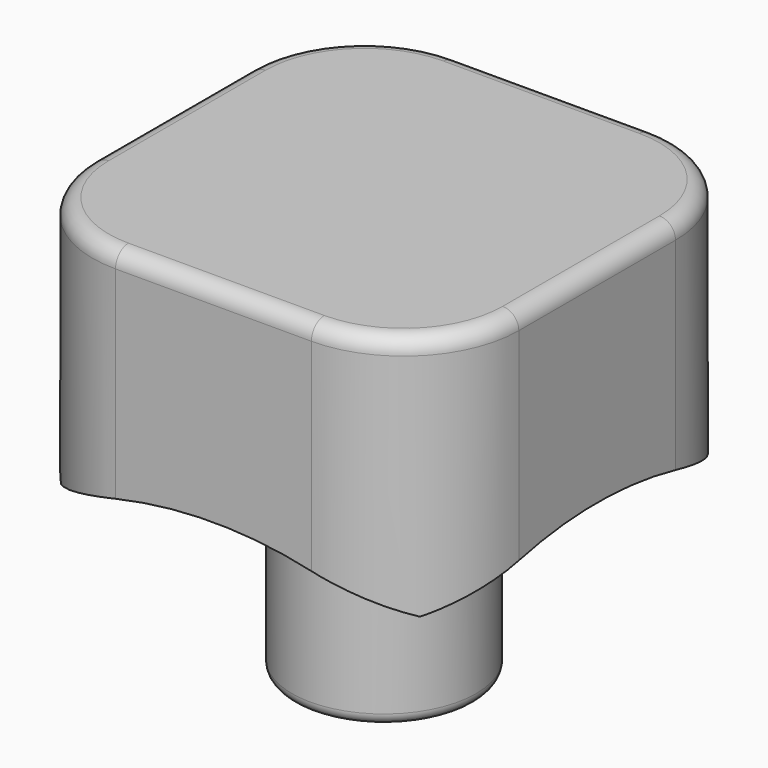
from build123d import *

# Parameters (mm, degrees)
F0_W         = 18.5
F0_H         = 11
F1_DEPTH     = 9.25
F2_DEPTH     = 9.25
F3_R         = 19
F5_DEPTH     = 25.4
F6_DEPTH     = 25.4
F4_R         = 19
F7_DEPTH     = 25.4
F8_DEPTH     = 25.4
F9_R         = 4
F10_DEPTH    = 3.45753
F11_DEPTH    = 7.5
F12_T1_DEPTH = 36
F13_R        = 0.7
F14_R        = 0.5


# Not quite as in the source:
# - a fillet or chamfer that OpenCascade refuses, or shapes differently, is made with other operations: its cross-section is extruded or revolved along the edge and cut away or added
# - a feature names something its author has since deleted; it is built from what else it names


with BuildPart() as f1:
    # F0 (on Front) → F1 (new body)
    with BuildSketch(Plane.XZ):
        Rectangle(F0_W, F0_H)
    extrude(amount=-F1_DEPTH)

    # F0 (on Front) → F2 (join)
    with BuildSketch(Plane.XZ):
        Rectangle(F0_W, F0_H)
    extrude(amount=F2_DEPTH)

    # F3 (on Front) → F5 (cut)
    with BuildSketch(Plane.XZ):
        with Locations((0, -22.5)):
            Circle(F3_R)
    extrude(amount=-F5_DEPTH, mode=Mode.SUBTRACT)

    # F3 (on Front) → F6 (cut)
    with BuildSketch(Plane.XZ):
        with Locations((0, -22.5)):
            Circle(F3_R)
    extrude(amount=F6_DEPTH, mode=Mode.SUBTRACT)

    # F4 (on Right) → F7 (cut)
    with BuildSketch(Plane.YZ):
        with Locations((0, -22.5)):
            Circle(F4_R)
    extrude(amount=-F7_DEPTH, mode=Mode.SUBTRACT)

    # F4 (on Right) → F8 (cut)
    with BuildSketch(Plane.YZ):
        with Locations((0, -22.5)):
            Circle(F4_R)
    extrude(amount=F8_DEPTH, mode=Mode.SUBTRACT)

    # F9 (on face) → F10 (join)
    with BuildSketch(Plane(origin=(0, 0, -5.5), x_dir=(1, 0, 0), z_dir=(0, 0, -1))):
        Circle(F9_R)
    extrude(amount=-F10_DEPTH)

    # F11 (add): a face of the model
    f11_faces = [f1.faces().sort_by_distance(p)[0] for p in [
        (0, 0, -5.5),
    ]]
    extrude(f11_faces, amount=F11_DEPTH)

    # F12: fillet of radius 5 on 4 edges, made by hand

    # F12_s2 → F12_t1 (cut)
    with BuildSketch(Plane.XY.offset(-18)):
        with BuildLine():
            ThreePointArc((-9.25, -4.25), (-7.7855339059, -7.7855339059), (-4.25, -9.25))
            Line((-4.25, -9.25), (-9.25, -9.25))
            Line((-9.25, -9.25), (-9.25, -4.25))
        make_face()
        with BuildLine():
            ThreePointArc((-4.25, 9.25), (-7.7855339059, 7.7855339059), (-9.25, 4.25))
            Line((-9.25, 4.25), (-9.25, 9.25))
            Line((-9.25, 9.25), (-4.25, 9.25))
        make_face()
        with BuildLine():
            ThreePointArc((9.25, 4.25), (7.7855339059, 7.7855339059), (4.25, 9.25))
            Line((4.25, 9.25), (9.25, 9.25))
            Line((9.25, 9.25), (9.25, 4.25))
        make_face()
        with BuildLine():
            ThreePointArc((9.25, -4.25), (7.7855339059, -7.7855339059), (4.25, -9.25))
            Line((4.25, -9.25), (9.25, -9.25))
            Line((9.25, -9.25), (9.25, -4.25))
        make_face()
    extrude(amount=F12_T1_DEPTH, mode=Mode.SUBTRACT)

    # F13
    f13_edges = [f1.edges().sort_by_distance(p)[0] for p in [
        (9.25, 0, 5.5),
        (7.785534, -7.785534, 5.5),
        (0, -9.25, 5.5),
        (-7.785534, -7.785534, 5.5),
        (-9.25, 0, 5.5),
        (-7.785534, 7.785534, 5.5),
        (0, 9.25, 5.5),
        (7.785534, 7.785534, 5.5),
    ]]
    fillet(f13_edges, radius=F13_R)

    # F14
    f14_edges = [f1.edges().sort_by_distance(p)[0] for p in [
        (-4, 0, -13),
    ]]
    fillet(f14_edges, radius=F14_R)


solid = f1.part
